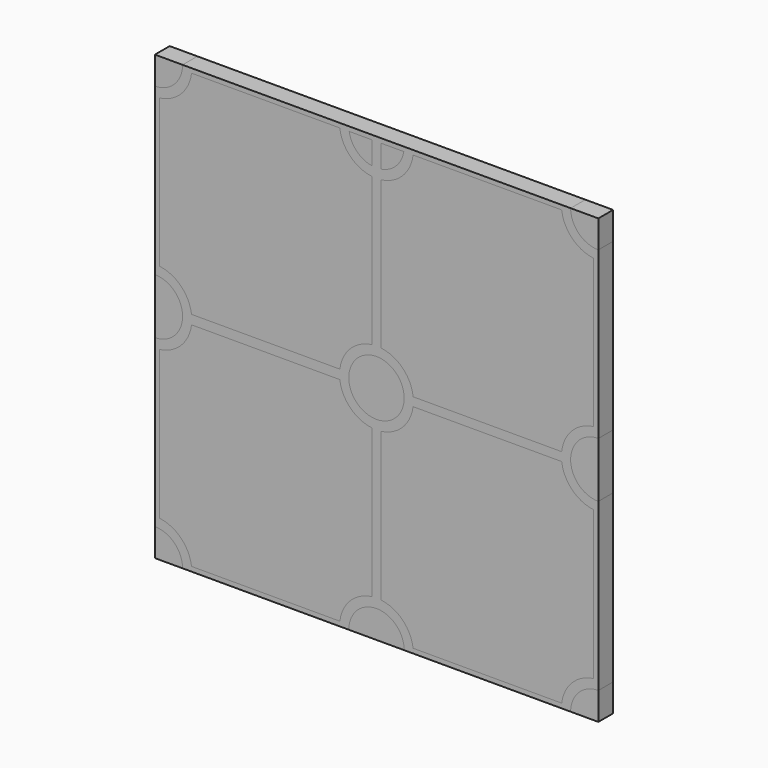
from build123d import *

# Parameters (mm, degrees)
F1_DEPTH = 6.349999999
F4_DEPTH = 6.35
F5_DEPTH = 6.3499998984
F6_DEPTH = 6.3499998984
F7_DEPTH = 6.3499998984


# Not quite as in the source:
# - a feature of the source that left no trace in its solid (it failed there, or was rolled back) is left out


with BuildPart() as f1:
    # F0 (on Front) → F1 (new body)
    with BuildSketch(Plane.XZ):
        with BuildLine():
            Line((-154.987726341, 108.204), (-162.8014844418, 108.204))
            Line((-162.8014844418, 108.204), (-162.8014844418, 100.3425733442))
            ThreePointArc((-162.8014844418, 100.3425733442), (-157.6333417325, 103.0196708129), (-154.987726341, 108.204))
        make_face()
        with BuildLine():
            Line((-151.781525698, 108.204), (-154.987726341, 108.204))
            ThreePointArc((-154.987726341, 108.204), (-157.6333417325, 103.0196708129), (-162.8014844418, 100.3425733442))
            Line((-162.8014844418, 100.3425733442), (-162.8014844418, 97.133959893))
            ThreePointArc((-162.8014844418, 97.133959893), (-155.3883922153, 100.7744768607), (-151.781525698, 108.204))
        make_face()
        with BuildLine():
            Line((-100.7829387975, 108.204), (-151.781525698, 108.204))
            ThreePointArc((-151.781525698, 108.204), (-155.3883922153, 100.7744768607), (-162.8014844418, 97.133959893))
            Line((-162.8014844418, 97.133959893), (-162.8014844418, 46.1790997877))
            ThreePointArc((-162.8014844418, 46.1790997877), (-155.4132877627, 42.563522416), (-151.7902119165, 35.179))
            Line((-151.7902119165, 35.179), (-100.7747638009, 35.179))
            ThreePointArc((-100.7747638009, 35.179), (-97.156319506, 42.5588931798), (-89.7764844418, 46.1774560004))
            Line((-89.7764844418, 46.1774560004), (-89.7764844418, 97.1361152558))
            ThreePointArc((-89.7764844418, 97.1361152558), (-97.1808433503, 100.7794778016), (-100.7829387975, 108.204))
        make_face()
        with BuildLine():
            Line((-97.5772493718, 108.204), (-100.7829387975, 108.204))
            ThreePointArc((-100.7829387975, 108.204), (-97.1808433503, 100.7794778016), (-89.7764844418, 97.1361152558))
            Line((-89.7764844418, 97.1361152558), (-89.7764844418, 100.3447788377))
            ThreePointArc((-89.7764844418, 100.3447788377), (-94.9362776614, 103.0243460565), (-97.5772493718, 108.204))
        make_face()
        with BuildLine():
            Line((-89.7764844418, 108.204), (-97.5772493718, 108.204))
            ThreePointArc((-97.5772493718, 108.204), (-94.9362776614, 103.0243460565), (-89.7764844418, 100.3447788377))
            Line((-89.7764844418, 100.3447788377), (-89.7764844418, 108.204))
        make_face()
    extrude(amount=-F1_DEPTH)


with BuildPart() as f4:
    # F0 (on Front) → F4 (new body)
    with BuildSketch(Plane.XZ):
        with BuildLine():
            Line((-100.7829387975, 108.204), (-151.781525698, 108.204))
            ThreePointArc((-151.781525698, 108.204), (-155.3883922153, 100.7744768607), (-162.8014844418, 97.133959893))
            Line((-162.8014844418, 97.133959893), (-162.8014844418, 46.1790997877))
            ThreePointArc((-162.8014844418, 46.1790997877), (-155.4132877627, 42.563522416), (-151.7902119165, 35.179))
            Line((-151.7902119165, 35.179), (-100.7747638009, 35.179))
            ThreePointArc((-100.7747638009, 35.179), (-97.156319506, 42.5588931798), (-89.7764844418, 46.1774560004))
            Line((-89.7764844418, 46.1774560004), (-89.7764844418, 97.1361152558))
            ThreePointArc((-89.7764844418, 97.1361152558), (-97.1808433503, 100.7794778016), (-100.7829387975, 108.204))
        make_face()
    extrude(amount=-F4_DEPTH)


with BuildPart() as f4b:
    # F0 (on Front) → F4, piece 2 (new body)
    with BuildSketch(Plane.XZ):
        with BuildLine():
            Line((-24.4689319785, 108.204), (-75.5690437445, 108.204))
            ThreePointArc((-75.5690437445, 108.204), (-79.180378369, 100.7701966336), (-86.6014844418, 97.1328411497))
            Line((-86.6014844418, 97.1328411497), (-86.6014844418, 46.1807299734))
            ThreePointArc((-86.6014844418, 46.1807299735), (-79.1422222135, 42.5051315593), (-75.5560500803, 35.0024662912))
            Line((-75.5560500803, 35.0024662912), (-24.481874521, 35.0024662912))
            ThreePointArc((-24.481874521, 35.0024662912), (-20.9003184276, 42.5004370686), (-13.4494844418, 46.1790485926))
            Line((-13.4494844418, 46.1790485926), (-13.4494844418, 97.1344713957))
            ThreePointArc((-13.4494844418, 97.1344713957), (-20.8622178353, 100.7748357215), (-24.4689319785, 108.204))
        make_face()
    extrude(amount=-F4_DEPTH)


with BuildPart() as f4c:
    # F0 (on Front) → F4, piece 3 (new body)
    with BuildSketch(Plane.XZ):
        with BuildLine():
            Line((-24.4639789262, 32.004401404), (-75.5739456025, 32.004401404))
            ThreePointArc((-75.5739456025, 32.004401404), (-79.1956642254, 24.5985239787), (-86.6014844418, 20.9766883744))
            Line((-86.6014844418, 20.9766883744), (-86.6014844418, -30.1330778462))
            ThreePointArc((-86.6014844418, -30.1330778462), (-79.2003661735, -33.7502139092), (-75.5756007032, -41.147598596))
            Line((-75.5756007032, -41.147598596), (-24.4623699509, -41.147598596))
            ThreePointArc((-24.4623699509, -41.147598596), (-20.8422369777, -33.7548460628), (-13.4494844418, -30.1347130949))
            Line((-13.4494844418, -30.1347130949), (-13.4494844418, 20.9783697553))
            ThreePointArc((-13.4494844418, 20.9783697553), (-20.8469041381, 24.6031909205), (-24.4639789262, 32.004401404))
        make_face()
    extrude(amount=-F4_DEPTH)


with BuildPart() as f4d:
    # F0 (on Front) → F4, piece 4 (new body)
    with BuildSketch(Plane.XZ):
        with BuildLine():
            Line((-100.7780369396, 32.004401404), (-151.7869387778, 32.004401404))
            ThreePointArc((-151.7869387778, 32.004401404), (-155.4040288349, 24.6031550064), (-162.8014844418, 20.9783185601))
            Line((-162.8014844418, 20.9783185601), (-162.8014844418, -30.1347080273))
            ThreePointArc((-162.8014844418, -30.1347080273), (-155.4087283563, -33.7548425102), (-151.7885938739, -41.147598596))
            Line((-151.7885938739, -41.147598596), (-100.7763818389, -41.147598596))
            ThreePointArc((-100.7763818389, -41.147598596), (-97.1155521358, -33.7143308752), (-89.6494844418, -30.1208678779))
            Line((-89.6494844418, -30.1208678779), (-89.6494844418, 20.9644784061))
            ThreePointArc((-89.6494844418, 20.9644784061), (-97.1202728718, 24.5626220718), (-100.7780369396, 32.004401404))
        make_face()
    extrude(amount=-F4_DEPTH)


with BuildPart() as f5:
    # F0 (on Front) → F5 (new body)
    with BuildSketch(Plane.XZ):
        with BuildLine():
            ThreePointArc((-154.9993787913, 35.179), (-157.6583808304, 40.3184866203), (-162.8014844418, 42.9704858296))
            Line((-162.8014844418, 42.9704858296), (-162.8014844418, 35.179))
            Line((-162.8014844418, 35.179), (-154.9993787913, 35.179))
        make_face()
        with BuildLine():
            ThreePointArc((-162.8014844418, 24.1869325182), (-157.6490642527, 26.8482485028), (-154.99498742, 32.004401404))
            Line((-154.99498742, 32.004401404), (-162.8014844418, 32.004401404))
            Line((-162.8014844418, 32.004401404), (-162.8014844418, 24.1869325182))
        make_face()
        with BuildLine():
            Line((-162.8014844418, 35.179), (-162.8014844418, 42.9704858296))
            ThreePointArc((-162.8014844418, 42.9704858296), (-163.5924443126, 43.0703449035), (-164.3889844418, 43.1037091739))
            Line((-164.3889844418, 43.1037091739), (-164.3889844418, 33.5787091739))
            Line((-164.3889844418, 33.5787091739), (-154.8639844418, 33.5787091739))
            ThreePointArc((-154.8639844418, 33.5787091739), (-154.897893387, 34.3817132769), (-154.9993787913, 35.179))
            Line((-154.9993787913, 35.179), (-162.8014844418, 35.179))
        make_face()
        with BuildLine():
            ThreePointArc((-154.99498742, 32.004401404), (-154.8967916858, 32.7888347005), (-154.8639844418, 33.5787091739))
            Line((-154.8639844418, 33.5787091739), (-164.3889844418, 33.5787091739))
            Line((-164.3889844418, 33.5787091739), (-164.3889844418, 24.0537091739))
            ThreePointArc((-164.3889844418, 24.0537091739), (-163.5924443126, 24.0870734444), (-162.8014844418, 24.1869325182))
            Line((-162.8014844418, 24.1869325182), (-162.8014844418, 32.004401404))
            Line((-162.8014844418, 32.004401404), (-154.99498742, 32.004401404))
        make_face()
    extrude(amount=-F5_DEPTH)


with BuildPart() as f5b:
    # F0 (on Front) → F5, piece 2 (new body)
    with BuildSketch(Plane.XZ):
        with BuildLine():
            ThreePointArc((-78.7580010039, 35.0024662912), (-81.3870446527, 40.259714249), (-86.6014844418, 42.9726728339))
            Line((-86.6014844418, 42.9726728339), (-86.6014844418, 35.2609418333))
            Line((-86.6014844418, 35.2609418333), (-86.6014844418, 35.0024662912))
            Line((-86.6014844418, 35.0024662912), (-78.7580010039, 35.0024662912))
        make_face()
        with BuildLine():
            Line((-89.7764844418, 35.179), (-89.7764844418, 42.9682803361))
            ThreePointArc((-89.7764844418, 42.9682803361), (-94.9112559328, 40.313828693), (-97.5655969215, 35.179))
            Line((-97.5655969215, 35.179), (-89.7764844418, 35.179))
        make_face()
        with BuildLine():
            Line((-89.6494844418, 32.004401404), (-97.5699882928, 32.004401404))
            ThreePointArc((-97.5699882928, 32.004401404), (-94.8749780887, 26.8075053949), (-89.6494844418, 24.1683721515))
            Line((-89.6494844418, 24.1683721515), (-89.6494844418, 32.004401404))
        make_face()
        with BuildLine():
            Line((-78.7819942492, 32.004401404), (-86.6014844418, 32.004401404))
            Line((-86.6014844418, 32.004401404), (-86.6014844418, 24.184745514))
            ThreePointArc((-86.6014844418, 24.184745514), (-81.440727821, 26.8435884432), (-78.7819942492, 32.004401404))
        make_face()
        with BuildLine():
            ThreePointArc((-86.6014844418, 42.9726728339), (-87.3860162275, 43.0708935606), (-88.175991271, 43.1037091739))
            Line((-88.175991271, 43.1037091739), (-88.175991271, 33.5787091739))
            Line((-88.175991271, 33.5787091739), (-86.6014844418, 35.2609418333))
            Line((-86.6014844418, 35.2609418333), (-86.6014844418, 42.9726728339))
        make_face()
        with BuildLine():
            Line((-86.6014844418, 35.2609418333), (-88.175991271, 33.5787091739))
            Line((-88.175991271, 33.5787091739), (-78.650991271, 33.5787091739))
            ThreePointArc((-78.650991271, 33.5787091739), (-78.6777813793, 34.2925956166), (-78.7580010039, 35.0024662912))
            Line((-78.7580010039, 35.0024662912), (-86.6014844418, 35.0024662912))
            Line((-86.6014844418, 35.0024662912), (-86.6014844418, 35.2609418333))
        make_face()
        with BuildLine():
            Line((-78.650991271, 33.5787091739), (-88.175991271, 33.5787091739))
            Line((-88.175991271, 33.5787091739), (-86.6014844418, 32.004401404))
            Line((-86.6014844418, 32.004401404), (-78.7819942492, 32.004401404))
            ThreePointArc((-78.7819942492, 32.004401404), (-78.6837985151, 32.7888347005), (-78.650991271, 33.5787091739))
        make_face()
        with BuildLine():
            Line((-86.6014844418, 32.004401404), (-88.175991271, 33.5787091739))
            Line((-88.175991271, 33.5787091739), (-88.175991271, 24.0537091739))
            ThreePointArc((-88.175991271, 24.0537091739), (-87.3860162275, 24.0865247872), (-86.6014844418, 24.184745514))
            Line((-86.6014844418, 24.184745514), (-86.6014844418, 32.004401404))
        make_face()
        with BuildLine():
            Line((-88.175991271, 24.0537091739), (-88.175991271, 33.5787091739))
            Line((-88.175991271, 33.5787091739), (-89.6494844418, 32.004401404))
            Line((-89.6494844418, 32.004401404), (-89.6494844418, 24.1683721515))
            ThreePointArc((-89.6494844418, 24.1683721515), (-88.9149651749, 24.0824181838), (-88.175991271, 24.0537091739))
        make_face()
        with BuildLine():
            ThreePointArc((-88.175991271, 43.1037091739), (-88.97909764, 43.0697915758), (-89.7764844418, 42.9682803361))
            Line((-89.7764844418, 42.9682803361), (-89.7764844418, 35.179))
            Line((-89.7764844418, 35.179), (-88.175991271, 33.5787091739))
            Line((-88.175991271, 33.5787091739), (-88.175991271, 43.1037091739))
        make_face()
        with BuildLine():
            Line((-89.7764844418, 35.179), (-97.5655969215, 35.179))
            ThreePointArc((-97.5655969215, 35.179), (-97.6670823258, 34.3817132769), (-97.700991271, 33.5787091739))
            Line((-97.700991271, 33.5787091739), (-88.175991271, 33.5787091739))
            Line((-88.175991271, 33.5787091739), (-89.7764844418, 35.179))
        make_face()
        with BuildLine():
            Line((-88.175991271, 33.5787091739), (-97.700991271, 33.5787091739))
            ThreePointArc((-97.700991271, 33.5787091739), (-97.668184027, 32.7888347005), (-97.5699882928, 32.004401404))
            Line((-97.5699882928, 32.004401404), (-89.6494844418, 32.004401404))
            Line((-89.6494844418, 32.004401404), (-88.175991271, 33.5787091739))
        make_face()
    extrude(amount=-F5_DEPTH)


with BuildPart() as f5c:
    # F0 (on Front) → F5, piece 3 (new body)
    with BuildSketch(Plane.XZ):
        with BuildLine():
            Line((-13.4494844418, 35.0024662912), (-13.4494844418, 42.9704858313))
            ThreePointArc((-13.4494844418, 42.9704858313), (-18.6555503637, 40.255017076), (-21.279974719, 35.0024662912))
            Line((-21.279974719, 35.0024662912), (-13.4494844418, 35.0024662912))
        make_face()
        with BuildLine():
            ThreePointArc((-11.861984452, 43.1037091739), (-12.658524576, 43.0703449039), (-13.4494844418, 42.9704858313))
            Line((-13.4494844418, 42.9704858313), (-13.4494844418, 35.0024662912))
            Line((-13.4494844418, 35.0024662912), (-21.279974719, 35.0024662912))
            ThreePointArc((-21.279974719, 35.0024662912), (-21.3601943437, 34.2925956166), (-21.386984452, 33.5787091739))
            Line((-21.386984452, 33.5787091739), (-11.861984452, 33.5787091739))
            Line((-11.861984452, 33.5787091739), (-11.861984452, 43.1037091739))
        make_face()
        with BuildLine():
            Line((-11.861984452, 33.5787091739), (-21.386984452, 33.5787091739))
            ThreePointArc((-21.386984452, 33.5787091739), (-21.3541772079, 32.7888347005), (-21.2559814738, 32.004401404))
            Line((-21.2559814738, 32.004401404), (-13.4494844418, 32.004401404))
            Line((-13.4494844418, 32.004401404), (-13.4494844418, 24.1869325165))
            ThreePointArc((-13.4494844418, 24.1869325165), (-12.658524576, 24.0870734439), (-11.861984452, 24.0537091739))
            Line((-11.861984452, 24.0537091739), (-11.861984452, 33.5787091739))
        make_face()
        with BuildLine():
            Line((-13.4494844418, 32.004401404), (-21.2559814738, 32.004401404))
            ThreePointArc((-21.2559814738, 32.004401404), (-18.6019046374, 26.8482484992), (-13.4494844418, 24.1869325165))
            Line((-13.4494844418, 24.1869325165), (-13.4494844418, 32.004401404))
        make_face()
    extrude(amount=-F5_DEPTH)


with BuildPart() as f5d:
    # F0 (on Front) → F5, piece 4 (new body)
    with BuildSketch(Plane.XZ):
        with BuildLine():
            Line((-13.4494844418, 108.204), (-21.2632425528, 108.204))
            ThreePointArc((-21.2632425528, 108.204), (-18.6176271576, 103.0196708092), (-13.4494844418, 100.3425733425))
            Line((-13.4494844418, 100.3425733425), (-13.4494844418, 108.204))
        make_face()
        with BuildLine():
            Line((-11.861984452, 109.7343499999), (-21.386984452, 109.7343499999))
            ThreePointArc((-21.386984452, 109.7343499999), (-21.3559985769, 108.9666776773), (-21.2632425528, 108.204))
            Line((-21.2632425528, 108.204), (-13.4494844418, 108.204))
            Line((-13.4494844418, 108.204), (-13.4494844418, 100.3425733425))
            ThreePointArc((-13.4494844418, 100.3425733425), (-12.658524576, 100.2427142699), (-11.861984452, 100.2093499999))
            Line((-11.861984452, 100.2093499999), (-11.861984452, 109.7343499999))
        make_face()
    extrude(amount=-F5_DEPTH)

    # F6 (add): a face of the model
    f6_faces = [f5d.faces().sort_by_distance(p)[0] for p in [
        (-15.9045200065, 0, 105.6918144454),
    ]]
    extrude(f6_faces, amount=-F6_DEPTH)


with BuildPart() as f5e:
    # F0 (on Front) → F5, piece 5 (new body)
    with BuildSketch(Plane.XZ):
        with BuildLine():
            ThreePointArc((-86.6014844418, 100.3403863399), (-81.4249943892, 103.014999875), (-78.7747331702, 108.204))
            Line((-78.7747331702, 108.204), (-86.6014844418, 108.204))
            Line((-86.6014844418, 108.204), (-86.6014844418, 100.3403863399))
        make_face()
        with BuildLine():
            Line((-89.7764844418, 108.204), (-97.5772493718, 108.204))
            ThreePointArc((-97.5772493718, 108.204), (-94.9362776614, 103.0243460565), (-89.7764844418, 100.3447788377))
            Line((-89.7764844418, 100.3447788377), (-89.7764844418, 108.204))
        make_face()
        with BuildLine():
            ThreePointArc((-97.700991271, 109.7343499999), (-97.670005396, 108.9666776773), (-97.5772493718, 108.204))
            Line((-97.5772493718, 108.204), (-89.7764844418, 108.204))
            Line((-89.7764844418, 108.204), (-89.7764844418, 100.3447788377))
            ThreePointArc((-89.7764844418, 100.3447788377), (-88.97909764, 100.243267598), (-88.175991271, 100.2093499999))
            Line((-88.175991271, 100.2093499999), (-88.175991271, 109.7343499999))
            Line((-88.175991271, 109.7343499999), (-97.700991271, 109.7343499999))
        make_face()
        with BuildLine():
            Line((-78.650991271, 109.7343499999), (-88.175991271, 109.7343499999))
            Line((-88.175991271, 109.7343499999), (-88.175991271, 100.2093499999))
            ThreePointArc((-88.175991271, 100.2093499999), (-87.3860162275, 100.2421656132), (-86.6014844418, 100.3403863399))
            Line((-86.6014844418, 100.3403863399), (-86.6014844418, 108.204))
            Line((-86.6014844418, 108.204), (-78.7747331702, 108.204))
            ThreePointArc((-78.7747331702, 108.204), (-78.6819771461, 108.9666776773), (-78.650991271, 109.7343499999))
        make_face()
    extrude(amount=-F5_DEPTH)


with BuildPart() as f5f:
    # F0 (on Front) → F5, piece 6 (new body)
    with BuildSketch(Plane.XZ):
        with BuildLine():
            Line((-154.987726341, 108.204), (-162.8014844418, 108.204))
            Line((-162.8014844418, 108.204), (-162.8014844418, 100.3425733442))
            ThreePointArc((-162.8014844418, 100.3425733442), (-157.6333417325, 103.0196708129), (-154.987726341, 108.204))
        make_face()
        with BuildLine():
            Line((-162.8014844418, 100.3425733442), (-162.8014844418, 108.204))
            Line((-162.8014844418, 108.204), (-164.3889844418, 108.204))
            Line((-164.3889844418, 108.204), (-164.3889844418, 100.2093499999))
            ThreePointArc((-164.3889844418, 100.2093499999), (-163.5924443126, 100.2427142703), (-162.8014844418, 100.3425733442))
        make_face()
        with BuildLine():
            Line((-164.3889844418, 108.204), (-162.8014844418, 108.204))
            Line((-162.8014844418, 108.204), (-154.987726341, 108.204))
            ThreePointArc((-154.987726341, 108.204), (-154.8949703168, 108.9666776773), (-154.8639844418, 109.7343499999))
            Line((-154.8639844418, 109.7343499999), (-164.3889844418, 109.7343499999))
            Line((-164.3889844418, 109.7343499999), (-164.3889844418, 108.204))
        make_face()
    extrude(amount=-F5_DEPTH)


with BuildPart() as f5g:
    # F0 (on Front) → F5, piece 7 (new body)
    with BuildSketch(Plane.XZ):
        with BuildLine():
            Line((-13.4494844418, -41.147598596), (-13.4494844418, -33.3433219376))
            ThreePointArc((-13.4494844418, -33.3433219376), (-18.5971765395, -35.9999065009), (-21.2537611078, -41.147598596))
            Line((-21.2537611078, -41.147598596), (-13.4494844418, -41.147598596))
        make_face()
        with BuildLine():
            Line((-11.861984452, -42.735098595), (-11.861984452, -33.210098595))
            ThreePointArc((-11.861984452, -33.210098595), (-12.658524576, -33.243462865), (-13.4494844418, -33.3433219376))
            Line((-13.4494844418, -33.3433219376), (-13.4494844418, -41.147598596))
            Line((-13.4494844418, -41.147598596), (-21.2537611078, -41.147598596))
            ThreePointArc((-21.2537611078, -41.147598596), (-21.3536201816, -41.9385584664), (-21.386984452, -42.735098595))
            Line((-21.386984452, -42.735098595), (-11.861984452, -42.735098595))
        make_face()
    extrude(amount=-F5_DEPTH)


with BuildPart() as f5h:
    # F0 (on Front) → F5, piece 8 (new body)
    with BuildSketch(Plane.XZ):
        with BuildLine():
            ThreePointArc((-78.7842146152, -41.147598596), (-81.4454591902, -35.9952497162), (-86.6014844418, -33.3411349351))
            Line((-86.6014844418, -33.3411349351), (-86.6014844418, -41.147598596))
            Line((-86.6014844418, -41.147598596), (-78.7842146152, -41.147598596))
        make_face()
        with BuildLine():
            Line((-89.6494844418, -41.147598596), (-89.6494844418, -33.3247615726))
            ThreePointArc((-89.6494844418, -33.3247615726), (-94.8702213892, -35.959192152), (-97.5677679269, -41.147598596))
            Line((-97.5677679269, -41.147598596), (-89.6494844418, -41.147598596))
        make_face()
        with BuildLine():
            ThreePointArc((-86.6014844418, -33.3411349351), (-87.3860162275, -33.2429142083), (-88.175991271, -33.210098595))
            Line((-88.175991271, -33.210098595), (-88.175991271, -42.735098595))
            Line((-88.175991271, -42.735098595), (-78.650991271, -42.735098595))
            ThreePointArc((-78.650991271, -42.735098595), (-78.6843555414, -41.9385584664), (-78.7842146152, -41.147598596))
            Line((-78.7842146152, -41.147598596), (-86.6014844418, -41.147598596))
            Line((-86.6014844418, -41.147598596), (-86.6014844418, -33.3411349351))
        make_face()
        with BuildLine():
            ThreePointArc((-88.175991271, -33.210098595), (-88.9149651749, -33.2388076049), (-89.6494844418, -33.3247615726))
            Line((-89.6494844418, -33.3247615726), (-89.6494844418, -41.147598596))
            Line((-89.6494844418, -41.147598596), (-97.5677679269, -41.147598596))
            ThreePointArc((-97.5677679269, -41.147598596), (-97.6676270006, -41.9385584664), (-97.700991271, -42.735098595))
            Line((-97.700991271, -42.735098595), (-88.175991271, -42.735098595))
            Line((-88.175991271, -42.735098595), (-88.175991271, -33.210098595))
        make_face()
    extrude(amount=-F5_DEPTH)


with BuildPart() as f5i:
    # F0 (on Front) → F5, piece 9 (new body)
    with BuildSketch(Plane.XZ):
        with BuildLine():
            ThreePointArc((-154.9972077859, -41.147598596), (-157.6537923506, -35.9999065046), (-162.8014844418, -33.3433219393))
            Line((-162.8014844418, -33.3433219393), (-162.8014844418, -41.147598596))
            Line((-162.8014844418, -41.147598596), (-154.9972077859, -41.147598596))
        make_face()
        with BuildLine():
            ThreePointArc((-162.8014844418, -33.3433219393), (-163.5924443126, -33.2434628655), (-164.3889844418, -33.210098595))
            Line((-164.3889844418, -33.210098595), (-164.3889844418, -42.735098595))
            Line((-164.3889844418, -42.735098595), (-154.8639844418, -42.735098595))
            ThreePointArc((-154.8639844418, -42.735098595), (-154.8973487122, -41.9385584664), (-154.9972077859, -41.147598596))
            Line((-154.9972077859, -41.147598596), (-162.8014844418, -41.147598596))
            Line((-162.8014844418, -41.147598596), (-162.8014844418, -33.3433219393))
        make_face()
    extrude(amount=-F5_DEPTH)


with BuildPart() as f7:
    # F0 (on Front) → F7 (new body)
    with BuildSketch(Plane.XZ):
        with BuildLine():
            ThreePointArc((-154.8639844418, 109.7343499999), (-154.8949703168, 108.9666776773), (-154.987726341, 108.204))
            Line((-154.987726341, 108.204), (-151.781525698, 108.204))
            ThreePointArc((-151.781525698, 108.204), (-151.7121412476, 108.9677772845), (-151.6889849498, 109.7343499999))
            Line((-151.6889849498, 109.7343499999), (-154.8639844418, 109.7343499999))
        make_face()
        with BuildLine():
            Line((-151.781525698, 108.204), (-154.987726341, 108.204))
            ThreePointArc((-154.987726341, 108.204), (-157.6333417325, 103.0196708129), (-162.8014844418, 100.3425733442))
            Line((-162.8014844418, 100.3425733442), (-162.8014844418, 97.133959893))
            ThreePointArc((-162.8014844418, 97.133959893), (-155.3883922153, 100.7744768607), (-151.781525698, 108.204))
        make_face()
        with BuildLine():
            Line((-162.8014844418, 97.133959893), (-162.8014844418, 100.3425733442))
            ThreePointArc((-162.8014844418, 100.3425733442), (-163.5924443126, 100.2427142703), (-164.3889844418, 100.2093499999))
            Line((-164.3889844418, 100.2093499999), (-164.3889844418, 97.0343505079))
            ThreePointArc((-164.3889844418, 97.0343505079), (-163.5936734523, 97.0592773166), (-162.8014844418, 97.133959893))
        make_face()
        with BuildLine():
            ThreePointArc((-151.6889849498, 109.7343499999), (-151.7121412476, 108.9677772845), (-151.781525698, 108.204))
            Line((-151.781525698, 108.204), (-100.7829387975, 108.204))
            ThreePointArc((-100.7829387975, 108.204), (-100.8523260393, 108.967777172), (-100.875483271, 109.7343499999))
            Line((-100.875483271, 109.7343499999), (-151.6889849498, 109.7343499999))
        make_face()
        with BuildLine():
            Line((-162.8014844418, 46.1790997877), (-162.8014844418, 97.133959893))
            ThreePointArc((-162.8014844418, 97.133959893), (-163.5936734523, 97.0592773166), (-164.3889844418, 97.0343505079))
            Line((-164.3889844418, 97.0343505079), (-164.3889844418, 46.2787091688))
            ThreePointArc((-164.3889844418, 46.2787091688), (-163.5936734525, 46.2537823611), (-162.8014844418, 46.1790997877))
        make_face()
        with BuildLine():
            ThreePointArc((-100.875483271, 109.7343499999), (-100.8523260393, 108.967777172), (-100.7829387975, 108.204))
            Line((-100.7829387975, 108.204), (-97.5772493718, 108.204))
            ThreePointArc((-97.5772493718, 108.204), (-97.670005396, 108.9666776773), (-97.700991271, 109.7343499999))
            Line((-97.700991271, 109.7343499999), (-100.875483271, 109.7343499999))
        make_face()
        with BuildLine():
            Line((-97.5772493718, 108.204), (-100.7829387975, 108.204))
            ThreePointArc((-100.7829387975, 108.204), (-97.1808433503, 100.7794778016), (-89.7764844418, 97.1361152558))
            Line((-89.7764844418, 97.1361152558), (-89.7764844418, 100.3447788377))
            ThreePointArc((-89.7764844418, 100.3447788377), (-94.9362776614, 103.0243460565), (-97.5772493718, 108.204))
        make_face()
        with BuildLine():
            ThreePointArc((-151.7902119165, 35.179), (-155.4132877627, 42.563522416), (-162.8014844418, 46.1790997877))
            Line((-162.8014844418, 46.1790997877), (-162.8014844418, 42.9704858296))
            ThreePointArc((-162.8014844418, 42.9704858296), (-157.6583808304, 40.3184866203), (-154.9993787913, 35.179))
            Line((-154.9993787913, 35.179), (-151.7902119165, 35.179))
        make_face()
        with BuildLine():
            Line((-162.8014844418, 42.9704858296), (-162.8014844418, 46.1790997877))
            ThreePointArc((-162.8014844418, 46.1790997877), (-163.5936734525, 46.2537823611), (-164.3889844418, 46.2787091688))
            Line((-164.3889844418, 46.2787091688), (-164.3889844418, 43.1037091739))
            ThreePointArc((-164.3889844418, 43.1037091739), (-163.5924443126, 43.0703449035), (-162.8014844418, 42.9704858296))
        make_face()
        with BuildLine():
            ThreePointArc((-97.700991271, 109.7343499999), (-97.670005396, 108.9666776773), (-97.5772493718, 108.204))
            Line((-97.5772493718, 108.204), (-89.7764844418, 108.204))
            Line((-89.7764844418, 108.204), (-89.7764844418, 100.3447788377))
            ThreePointArc((-89.7764844418, 100.3447788377), (-88.97909764, 100.243267598), (-88.175991271, 100.2093499999))
            Line((-88.175991271, 100.2093499999), (-88.175991271, 109.7343499999))
            Line((-88.175991271, 109.7343499999), (-97.700991271, 109.7343499999))
        make_face()
        with BuildLine():
            ThreePointArc((-88.175991271, 97.0348579999), (-88.9778377996, 97.0601975942), (-89.7764844418, 97.1361152558))
            Line((-89.7764844418, 97.1361152558), (-89.7764844418, 46.1774560004))
            ThreePointArc((-89.7764844418, 46.1774560004), (-88.9778376707, 46.2533706029), (-88.175991271, 46.2787091734))
            Line((-88.175991271, 46.2787091734), (-88.175991271, 97.0348579999))
        make_face()
        with BuildLine():
            Line((-89.7764844418, 100.3447788377), (-89.7764844418, 97.1361152558))
            ThreePointArc((-89.7764844418, 97.1361152558), (-88.9778377996, 97.0601975942), (-88.175991271, 97.0348579999))
            Line((-88.175991271, 97.0348579999), (-88.175991271, 100.2093499999))
            ThreePointArc((-88.175991271, 100.2093499999), (-88.97909764, 100.243267598), (-89.7764844418, 100.3447788377))
        make_face()
        with BuildLine():
            ThreePointArc((-151.6889844468, 33.5787091739), (-151.7143165787, 34.3804537917), (-151.7902119165, 35.179))
            Line((-151.7902119165, 35.179), (-154.9993787913, 35.179))
            ThreePointArc((-154.9993787913, 35.179), (-154.897893387, 34.3817132769), (-154.8639844418, 33.5787091739))
            Line((-154.8639844418, 33.5787091739), (-151.6889844468, 33.5787091739))
        make_face()
        with BuildLine():
            Line((-100.7747638009, 35.179), (-151.7902119165, 35.179))
            ThreePointArc((-151.7902119165, 35.179), (-151.7143165787, 34.3804537917), (-151.6889844468, 33.5787091739))
            Line((-151.6889844468, 33.5787091739), (-100.8759912705, 33.5787091739))
            ThreePointArc((-100.8759912705, 33.5787091739), (-100.8506591387, 34.3804537917), (-100.7747638009, 35.179))
        make_face()
        with BuildLine():
            ThreePointArc((-75.5690437445, 108.204), (-75.4996565028, 108.967777172), (-75.476499271, 109.7343499999))
            Line((-75.476499271, 109.7343499999), (-78.650991271, 109.7343499999))
            ThreePointArc((-78.650991271, 109.7343499999), (-78.6819771461, 108.9666776773), (-78.7747331702, 108.204))
            Line((-78.7747331702, 108.204), (-75.5690437445, 108.204))
        make_face()
        with BuildLine():
            Line((-24.561476452, 109.7343499999), (-75.476499271, 109.7343499999))
            ThreePointArc((-75.476499271, 109.7343499999), (-75.4996565028, 108.967777172), (-75.5690437445, 108.204))
            Line((-75.5690437445, 108.204), (-24.4689319785, 108.204))
            ThreePointArc((-24.4689319785, 108.204), (-24.5383192202, 108.967777172), (-24.561476452, 109.7343499999))
        make_face()
        with BuildLine():
            ThreePointArc((-88.175991271, 46.2787091734), (-88.9778376707, 46.2533706029), (-89.7764844418, 46.1774560004))
            Line((-89.7764844418, 46.1774560004), (-89.7764844418, 42.9682803361))
            ThreePointArc((-89.7764844418, 42.9682803361), (-88.97909764, 43.0697915758), (-88.175991271, 43.1037091739))
            Line((-88.175991271, 43.1037091739), (-88.175991271, 46.2787091734))
        make_face()
        with BuildLine():
            Line((-89.7764844418, 42.9682803361), (-89.7764844418, 46.1774560004))
            ThreePointArc((-89.7764844418, 46.1774560004), (-97.156319506, 42.5588931798), (-100.7747638009, 35.179))
            Line((-100.7747638009, 35.179), (-97.5655969215, 35.179))
            ThreePointArc((-97.5655969215, 35.179), (-94.9112559328, 40.313828693), (-89.7764844418, 42.9682803361))
        make_face()
        with BuildLine():
            ThreePointArc((-86.6014844418, 97.1328411497), (-87.3872149319, 97.0593774577), (-88.175991271, 97.0348579999))
            Line((-88.175991271, 97.0348579999), (-88.175991271, 46.2787091734))
            ThreePointArc((-88.175991271, 46.2787091734), (-87.3872150545, 46.2541907059), (-86.6014844418, 46.1807299735))
            Line((-86.6014844418, 46.1807299734), (-86.6014844418, 97.1328411497))
        make_face()
        with BuildLine():
            Line((-88.175991271, 100.2093499999), (-88.175991271, 97.0348579999))
            ThreePointArc((-88.175991271, 97.0348579999), (-87.3872149319, 97.0593774577), (-86.6014844418, 97.1328411497))
            Line((-86.6014844418, 97.1328411497), (-86.6014844418, 100.3403863399))
            ThreePointArc((-86.6014844418, 100.3403863399), (-87.3860162275, 100.2421656132), (-88.175991271, 100.2093499999))
        make_face()
        with BuildLine():
            Line((-97.5655969215, 35.179), (-100.7747638009, 35.179))
            ThreePointArc((-100.7747638009, 35.179), (-100.8506591387, 34.3804537917), (-100.8759912705, 33.5787091739))
            Line((-100.8759912705, 33.5787091739), (-97.700991271, 33.5787091739))
            ThreePointArc((-97.700991271, 33.5787091739), (-97.6670823258, 34.3817132769), (-97.5655969215, 35.179))
        make_face()
        with BuildLine():
            ThreePointArc((-151.7869387778, 32.004401404), (-151.7134966851, 32.7900330672), (-151.6889844468, 33.5787091739))
            Line((-151.6889844468, 33.5787091739), (-154.8639844418, 33.5787091739))
            ThreePointArc((-154.8639844418, 33.5787091739), (-154.8967916858, 32.7888347005), (-154.99498742, 32.004401404))
            Line((-154.99498742, 32.004401404), (-151.7869387778, 32.004401404))
        make_face()
        with BuildLine():
            Line((-100.8759912705, 33.5787091739), (-151.6889844468, 33.5787091739))
            ThreePointArc((-151.6889844468, 33.5787091739), (-151.7134966851, 32.7900330672), (-151.7869387778, 32.004401404))
            Line((-151.7869387778, 32.004401404), (-100.7780369396, 32.004401404))
            ThreePointArc((-100.7780369396, 32.004401404), (-100.8514790323, 32.7900330672), (-100.8759912705, 33.5787091739))
        make_face()
        with BuildLine():
            Line((-78.650991271, 109.7343499999), (-88.175991271, 109.7343499999))
            Line((-88.175991271, 109.7343499999), (-88.175991271, 100.2093499999))
            ThreePointArc((-88.175991271, 100.2093499999), (-87.3860162275, 100.2421656132), (-86.6014844418, 100.3403863399))
            Line((-86.6014844418, 100.3403863399), (-86.6014844418, 108.204))
            Line((-86.6014844418, 108.204), (-78.7747331702, 108.204))
            ThreePointArc((-78.7747331702, 108.204), (-78.6819771461, 108.9666776773), (-78.650991271, 109.7343499999))
        make_face()
        with BuildLine():
            Line((-21.386984452, 109.7343499999), (-24.561476452, 109.7343499999))
            ThreePointArc((-24.561476452, 109.7343499999), (-24.5383192202, 108.967777172), (-24.4689319785, 108.204))
            Line((-24.4689319785, 108.204), (-21.2632425528, 108.204))
            ThreePointArc((-21.2632425528, 108.204), (-21.3559985769, 108.9666776773), (-21.386984452, 109.7343499999))
        make_face()
        with BuildLine():
            ThreePointArc((-86.6014844418, 97.1328411497), (-79.180378369, 100.7701966336), (-75.5690437445, 108.204))
            Line((-75.5690437445, 108.204), (-78.7747331702, 108.204))
            ThreePointArc((-78.7747331702, 108.204), (-81.4249943892, 103.014999875), (-86.6014844418, 100.3403863399))
            Line((-86.6014844418, 100.3403863399), (-86.6014844418, 97.1328411497))
        make_face()
        with BuildLine():
            ThreePointArc((-86.6014844418, 46.1807299735), (-87.3872150545, 46.2541907059), (-88.175991271, 46.2787091734))
            Line((-88.175991271, 46.2787091734), (-88.175991271, 43.1037091739))
            ThreePointArc((-88.175991271, 43.1037091739), (-87.3860162275, 43.0708935606), (-86.6014844418, 42.9726728339))
            Line((-86.6014844418, 42.9726728339), (-86.6014844418, 46.1807299734))
        make_face()
        with BuildLine():
            Line((-97.700991271, 33.5787091739), (-100.8759912705, 33.5787091739))
            ThreePointArc((-100.8759912705, 33.5787091739), (-100.8514790323, 32.7900330672), (-100.7780369396, 32.004401404))
            Line((-100.7780369396, 32.004401404), (-97.5699882928, 32.004401404))
            ThreePointArc((-97.5699882928, 32.004401404), (-97.668184027, 32.7888347005), (-97.700991271, 33.5787091739))
        make_face()
        with BuildLine():
            ThreePointArc((-162.8014844418, 20.9783185601), (-155.4040288349, 24.6031550064), (-151.7869387778, 32.004401404))
            Line((-151.7869387778, 32.004401404), (-154.99498742, 32.004401404))
            ThreePointArc((-154.99498742, 32.004401404), (-157.6490642527, 26.8482485028), (-162.8014844418, 24.1869325182))
            Line((-162.8014844418, 24.1869325182), (-162.8014844418, 20.9783185601))
        make_face()
        with BuildLine():
            ThreePointArc((-162.8014844418, 20.9783185601), (-163.5936734525, 20.9036359867), (-164.3889844418, 20.878709179))
            Line((-164.3889844418, 20.878709179), (-164.3889844418, -30.0350986458))
            ThreePointArc((-164.3889844418, -30.0350986458), (-163.5936734525, -30.0600254536), (-162.8014844418, -30.1347080273))
            Line((-162.8014844418, -30.1347080273), (-162.8014844418, 20.9783185601))
        make_face()
        with BuildLine():
            Line((-164.3889844418, 24.0537091739), (-164.3889844418, 20.878709179))
            ThreePointArc((-164.3889844418, 20.878709179), (-163.5936734525, 20.9036359867), (-162.8014844418, 20.9783185601))
            Line((-162.8014844418, 20.9783185601), (-162.8014844418, 24.1869325182))
            ThreePointArc((-162.8014844418, 24.1869325182), (-163.5924443126, 24.0870734444), (-164.3889844418, 24.0537091739))
        make_face()
        with BuildLine():
            Line((-21.2632425528, 108.204), (-24.4689319785, 108.204))
            ThreePointArc((-24.4689319785, 108.204), (-20.8622178353, 100.7748357215), (-13.4494844418, 97.1344713957))
            Line((-13.4494844418, 97.1344713957), (-13.4494844418, 100.3425733425))
            ThreePointArc((-13.4494844418, 100.3425733425), (-18.6176271576, 103.0196708092), (-21.2632425528, 108.204))
        make_face()
        with BuildLine():
            ThreePointArc((-75.5560500803, 35.0024662912), (-79.1422222135, 42.5051315593), (-86.6014844418, 46.1807299735))
            Line((-86.6014844418, 46.1807299734), (-86.6014844418, 42.9726728339))
            ThreePointArc((-86.6014844418, 42.9726728339), (-81.3870446527, 40.259714249), (-78.7580010039, 35.0024662912))
            Line((-78.7580010039, 35.0024662912), (-75.5560500803, 35.0024662912))
        make_face()
        with BuildLine():
            Line((-97.5699882928, 32.004401404), (-100.7780369396, 32.004401404))
            ThreePointArc((-100.7780369396, 32.004401404), (-97.1202728718, 24.5626220718), (-89.6494844418, 20.9644784061))
            Line((-89.6494844418, 20.9644784061), (-89.6494844418, 24.1683721515))
            ThreePointArc((-89.6494844418, 24.1683721515), (-94.8749780887, 26.8075053949), (-97.5699882928, 32.004401404))
        make_face()
        with BuildLine():
            ThreePointArc((-162.8014844418, -30.1347080273), (-163.5936734525, -30.0600254536), (-164.3889844418, -30.0350986458))
            Line((-164.3889844418, -30.0350986458), (-164.3889844418, -33.210098595))
            ThreePointArc((-164.3889844418, -33.210098595), (-163.5924443126, -33.2434628655), (-162.8014844418, -33.3433219393))
            Line((-162.8014844418, -33.3433219393), (-162.8014844418, -30.1347080273))
        make_face()
        with BuildLine():
            ThreePointArc((-11.861984452, 97.0348579999), (-12.6572955619, 97.0597858142), (-13.4494844418, 97.1344713957))
            Line((-13.4494844418, 97.1344713957), (-13.4494844418, 46.1790485926))
            ThreePointArc((-13.4494844418, 46.1790485926), (-12.6572954487, 46.2537314659), (-11.861984452, 46.2786583739))
            Line((-11.861984452, 46.2786583739), (-11.861984452, 97.0348579999))
        make_face()
        with BuildLine():
            Line((-13.4494844418, 100.3425733425), (-13.4494844418, 97.1344713957))
            ThreePointArc((-13.4494844418, 97.1344713957), (-12.6572955619, 97.0597858142), (-11.861984452, 97.0348579999))
            Line((-11.861984452, 97.0348579999), (-11.861984452, 100.2093499999))
            ThreePointArc((-11.861984452, 100.2093499999), (-12.658524576, 100.2427142699), (-13.4494844418, 100.3425733425))
        make_face()
        with BuildLine():
            ThreePointArc((-75.4759912715, 33.5787091739), (-75.4960217698, 34.2917122843), (-75.5560500803, 35.0024662912))
            Line((-75.5560500803, 35.0024662912), (-78.7580010039, 35.0024662912))
            ThreePointArc((-78.7580010039, 35.0024662912), (-78.6777813793, 34.2925956166), (-78.650991271, 33.5787091739))
            Line((-78.650991271, 33.5787091739), (-75.4759912715, 33.5787091739))
        make_face()
        with BuildLine():
            Line((-24.481874521, 35.0024662912), (-75.5560500803, 35.0024662912))
            ThreePointArc((-75.5560500803, 35.0024662912), (-75.4960217698, 34.2917122843), (-75.4759912715, 33.5787091739))
            Line((-75.4759912715, 33.5787091739), (-24.561933652, 33.5787091739))
            ThreePointArc((-24.561933652, 33.5787091739), (-24.5419030729, 34.2917122934), (-24.481874521, 35.0024662912))
        make_face()
        with BuildLine():
            ThreePointArc((-88.175991271, 20.8787091744), (-88.9139849169, 20.9001696143), (-89.6494844418, 20.9644784061))
            Line((-89.6494844418, 20.9644784061), (-89.6494844418, -30.1208678779))
            ThreePointArc((-89.6494844418, -30.1208678779), (-88.9139849169, -30.0565590857), (-88.175991271, -30.0350986458))
            Line((-88.175991271, -30.0350986458), (-88.175991271, 20.8787091744))
        make_face()
        with BuildLine():
            Line((-89.6494844418, 24.1683721515), (-89.6494844418, 20.9644784061))
            ThreePointArc((-89.6494844418, 20.9644784061), (-88.9139849169, 20.9001696143), (-88.175991271, 20.8787091744))
            Line((-88.175991271, 20.8787091744), (-88.175991271, 24.0537091739))
            ThreePointArc((-88.175991271, 24.0537091739), (-88.9149651749, 24.0824181838), (-89.6494844418, 24.1683721515))
        make_face()
        with BuildLine():
            ThreePointArc((-151.7885938739, -41.147598596), (-155.4087283563, -33.7548425102), (-162.8014844418, -30.1347080273))
            Line((-162.8014844418, -30.1347080273), (-162.8014844418, -33.3433219393))
            ThreePointArc((-162.8014844418, -33.3433219393), (-157.6537923506, -35.9999065046), (-154.9972077859, -41.147598596))
            Line((-154.9972077859, -41.147598596), (-151.7885938739, -41.147598596))
        make_face()
        with BuildLine():
            ThreePointArc((-11.861984452, 46.2786583739), (-12.6572954487, 46.2537314659), (-13.4494844418, 46.1790485926))
            Line((-13.4494844418, 46.1790485926), (-13.4494844418, 42.9704858313))
            ThreePointArc((-13.4494844418, 42.9704858313), (-12.658524576, 43.0703449039), (-11.861984452, 43.1037091739))
            Line((-11.861984452, 43.1037091739), (-11.861984452, 46.2786583739))
        make_face()
        with BuildLine():
            Line((-13.4494844418, 42.9704858313), (-13.4494844418, 46.1790485926))
            ThreePointArc((-13.4494844418, 46.1790485926), (-20.9003184276, 42.5004370686), (-24.481874521, 35.0024662912))
            Line((-24.481874521, 35.0024662912), (-21.279974719, 35.0024662912))
            ThreePointArc((-21.279974719, 35.0024662912), (-18.6555503637, 40.255017076), (-13.4494844418, 42.9704858313))
        make_face()
        with BuildLine():
            Line((-75.4759912715, 33.5787091739), (-78.650991271, 33.5787091739))
            ThreePointArc((-78.650991271, 33.5787091739), (-78.6837985151, 32.7888347005), (-78.7819942492, 32.004401404))
            Line((-78.7819942492, 32.004401404), (-75.5739456025, 32.004401404))
            ThreePointArc((-75.5739456025, 32.004401404), (-75.5005035098, 32.7900330672), (-75.4759912715, 33.5787091739))
        make_face()
        with BuildLine():
            ThreePointArc((-86.6014844418, 24.184745514), (-87.3860162275, 24.0865247872), (-88.175991271, 24.0537091739))
            Line((-88.175991271, 24.0537091739), (-88.175991271, 20.8787091744))
            ThreePointArc((-88.175991271, 20.8787091744), (-87.3872150545, 20.9032276419), (-86.6014844418, 20.9766883744))
            Line((-86.6014844418, 20.9766883744), (-86.6014844418, 24.184745514))
        make_face()
        with BuildLine():
            Line((-21.279974719, 35.0024662912), (-24.481874521, 35.0024662912))
            ThreePointArc((-24.481874521, 35.0024662912), (-24.5419030729, 34.2917122934), (-24.561933652, 33.5787091739))
            Line((-24.561933652, 33.5787091739), (-21.386984452, 33.5787091739))
            ThreePointArc((-21.386984452, 33.5787091739), (-21.3601943437, 34.2925956166), (-21.279974719, 35.0024662912))
        make_face()
        with BuildLine():
            Line((-24.561933652, 33.5787091739), (-75.4759912715, 33.5787091739))
            ThreePointArc((-75.4759912715, 33.5787091739), (-75.5005035098, 32.7900330672), (-75.5739456025, 32.004401404))
            Line((-75.5739456025, 32.004401404), (-24.4639789262, 32.004401404))
            ThreePointArc((-24.4639789262, 32.004401404), (-24.5374213147, 32.7900330549), (-24.561933652, 33.5787091739))
        make_face()
        with BuildLine():
            ThreePointArc((-88.175991271, -30.0350986458), (-88.9139849169, -30.0565590857), (-89.6494844418, -30.1208678779))
            Line((-89.6494844418, -30.1208678779), (-89.6494844418, -33.3247615726))
            ThreePointArc((-89.6494844418, -33.3247615726), (-88.9149651749, -33.2388076049), (-88.175991271, -33.210098595))
            Line((-88.175991271, -33.210098595), (-88.175991271, -30.0350986458))
        make_face()
        with BuildLine():
            Line((-89.6494844418, -33.3247615726), (-89.6494844418, -30.1208678779))
            ThreePointArc((-89.6494844418, -30.1208678779), (-97.1155521358, -33.7143308752), (-100.7763818389, -41.147598596))
            Line((-100.7763818389, -41.147598596), (-97.5677679269, -41.147598596))
            ThreePointArc((-97.5677679269, -41.147598596), (-94.8702213892, -35.959192152), (-89.6494844418, -33.3247615726))
        make_face()
        with BuildLine():
            ThreePointArc((-86.6014844418, 20.9766883744), (-87.3872150545, 20.9032276419), (-88.175991271, 20.8787091744))
            Line((-88.175991271, 20.8787091744), (-88.175991271, -30.0350986458))
            ThreePointArc((-88.175991271, -30.0350986458), (-87.3872150545, -30.0596171134), (-86.6014844418, -30.1330778462))
            Line((-86.6014844418, -30.1330778462), (-86.6014844418, 20.9766883744))
        make_face()
        with BuildLine():
            ThreePointArc((-151.6889844926, -42.735098595), (-151.7139113003, -41.9397876062), (-151.7885938739, -41.147598596))
            Line((-151.7885938739, -41.147598596), (-154.9972077859, -41.147598596))
            ThreePointArc((-154.9972077859, -41.147598596), (-154.8973487122, -41.9385584664), (-154.8639844418, -42.735098595))
            Line((-154.8639844418, -42.735098595), (-151.6889844926, -42.735098595))
        make_face()
        with BuildLine():
            Line((-100.7763818389, -41.147598596), (-151.7885938739, -41.147598596))
            ThreePointArc((-151.7885938739, -41.147598596), (-151.7139113003, -41.9397876062), (-151.6889844926, -42.735098595))
            Line((-151.6889844926, -42.735098595), (-100.8759912202, -42.735098595))
            ThreePointArc((-100.8759912202, -42.735098595), (-100.8510644125, -41.9397876062), (-100.7763818389, -41.147598596))
        make_face()
        with BuildLine():
            Line((-75.5739456025, 32.004401404), (-78.7819942492, 32.004401404))
            ThreePointArc((-78.7819942492, 32.004401404), (-81.440727821, 26.8435884432), (-86.6014844418, 24.184745514))
            Line((-86.6014844418, 24.184745514), (-86.6014844418, 20.9766883744))
            ThreePointArc((-86.6014844418, 20.9766883744), (-79.1956642254, 24.5985239787), (-75.5739456025, 32.004401404))
        make_face()
        with BuildLine():
            Line((-21.386984452, 33.5787091739), (-24.561933652, 33.5787091739))
            ThreePointArc((-24.561933652, 33.5787091739), (-24.5374213147, 32.7900330549), (-24.4639789262, 32.004401404))
            Line((-24.4639789262, 32.004401404), (-21.2559814738, 32.004401404))
            ThreePointArc((-21.2559814738, 32.004401404), (-21.3541772079, 32.7888347005), (-21.386984452, 33.5787091739))
        make_face()
        with BuildLine():
            ThreePointArc((-86.6014844418, -30.1330778462), (-87.3872150545, -30.0596171134), (-88.175991271, -30.0350986458))
            Line((-88.175991271, -30.0350986458), (-88.175991271, -33.210098595))
            ThreePointArc((-88.175991271, -33.210098595), (-87.3860162275, -33.2429142083), (-86.6014844418, -33.3411349351))
            Line((-86.6014844418, -33.3411349351), (-86.6014844418, -30.1330778462))
        make_face()
        with BuildLine():
            Line((-97.5677679269, -41.147598596), (-100.7763818389, -41.147598596))
            ThreePointArc((-100.7763818389, -41.147598596), (-100.8510644125, -41.9397876062), (-100.8759912202, -42.735098595))
            Line((-100.8759912202, -42.735098595), (-97.700991271, -42.735098595))
            ThreePointArc((-97.700991271, -42.735098595), (-97.6676270006, -41.9385584664), (-97.5677679269, -41.147598596))
        make_face()
        with BuildLine():
            Line((-21.2559814738, 32.004401404), (-24.4639789262, 32.004401404))
            ThreePointArc((-24.4639789262, 32.004401404), (-20.8469041381, 24.6031909205), (-13.4494844418, 20.9783697553))
            Line((-13.4494844418, 20.9783697553), (-13.4494844418, 24.1869325165))
            ThreePointArc((-13.4494844418, 24.1869325165), (-18.6019046374, 26.8482484992), (-21.2559814738, 32.004401404))
        make_face()
        with BuildLine():
            ThreePointArc((-75.5756007032, -41.147598596), (-79.2003661735, -33.7502139092), (-86.6014844418, -30.1330778462))
            Line((-86.6014844418, -30.1330778462), (-86.6014844418, -33.3411349351))
            ThreePointArc((-86.6014844418, -33.3411349351), (-81.4454591902, -35.9952497162), (-78.7842146152, -41.147598596))
            Line((-78.7842146152, -41.147598596), (-75.5756007032, -41.147598596))
        make_face()
        with BuildLine():
            ThreePointArc((-13.4494844418, 20.9783697553), (-12.6572954487, 20.903686882), (-11.861984452, 20.8787599739))
            Line((-11.861984452, 20.8787599739), (-11.861984452, 24.0537091739))
            ThreePointArc((-11.861984452, 24.0537091739), (-12.658524576, 24.0870734439), (-13.4494844418, 24.1869325165))
            Line((-13.4494844418, 24.1869325165), (-13.4494844418, 20.9783697553))
        make_face()
        with BuildLine():
            Line((-11.861984452, -30.035103675), (-11.861984452, 20.8787599739))
            ThreePointArc((-11.861984452, 20.8787599739), (-12.6572954487, 20.903686882), (-13.4494844418, 20.9783697553))
            Line((-13.4494844418, 20.9783697553), (-13.4494844418, -30.1347130949))
            ThreePointArc((-13.4494844418, -30.1347130949), (-12.6572954374, -30.0600304925), (-11.861984452, -30.035103675))
        make_face()
        with BuildLine():
            ThreePointArc((-75.4759913218, -42.735098595), (-75.5009181296, -41.9397876062), (-75.5756007032, -41.147598596))
            Line((-75.5756007032, -41.147598596), (-78.7842146152, -41.147598596))
            ThreePointArc((-78.7842146152, -41.147598596), (-78.6843555414, -41.9385584664), (-78.650991271, -42.735098595))
            Line((-78.650991271, -42.735098595), (-75.4759913218, -42.735098595))
        make_face()
        with BuildLine():
            Line((-24.4623699509, -41.147598596), (-75.5756007032, -41.147598596))
            ThreePointArc((-75.5756007032, -41.147598596), (-75.5009181296, -41.9397876062), (-75.4759913218, -42.735098595))
            Line((-75.4759913218, -42.735098595), (-24.561979372, -42.735098595))
            ThreePointArc((-24.561979372, -42.735098595), (-24.5370525542, -41.939787605), (-24.4623699509, -41.147598596))
        make_face()
        with BuildLine():
            Line((-11.861984452, -33.210098595), (-11.861984452, -30.035103675))
            ThreePointArc((-11.861984452, -30.035103675), (-12.6572954374, -30.0600304925), (-13.4494844418, -30.1347130949))
            Line((-13.4494844418, -30.1347130949), (-13.4494844418, -33.3433219376))
            ThreePointArc((-13.4494844418, -33.3433219376), (-12.658524576, -33.243462865), (-11.861984452, -33.210098595))
        make_face()
        with BuildLine():
            Line((-13.4494844418, -33.3433219376), (-13.4494844418, -30.1347130949))
            ThreePointArc((-13.4494844418, -30.1347130949), (-20.8422369777, -33.7548460628), (-24.4623699509, -41.147598596))
            Line((-24.4623699509, -41.147598596), (-21.2537611078, -41.147598596))
            ThreePointArc((-21.2537611078, -41.147598596), (-18.5971765395, -35.9999065009), (-13.4494844418, -33.3433219376))
        make_face()
        with BuildLine():
            Line((-21.2537611078, -41.147598596), (-24.4623699509, -41.147598596))
            ThreePointArc((-24.4623699509, -41.147598596), (-24.5370525542, -41.939787605), (-24.561979372, -42.735098595))
            Line((-24.561979372, -42.735098595), (-21.386984452, -42.735098595))
            ThreePointArc((-21.386984452, -42.735098595), (-21.3536201816, -41.9385584664), (-21.2537611078, -41.147598596))
        make_face()
    extrude(amount=-F7_DEPTH)


solid = Compound([f4.part, f4b.part, f4c.part, f4d.part, f5.part, f5b.part, f5c.part, f5d.part, f5e.part, f5f.part, f5g.part, f5h.part, f5i.part, f7.part])
